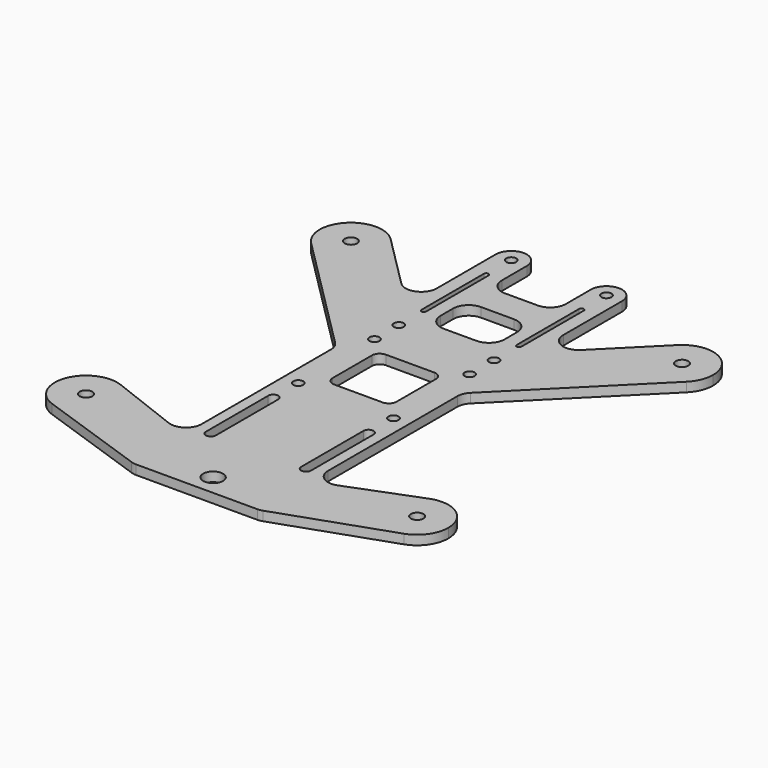
from build123d import *

# Parameters (mm, degrees)
F0_R      = 2
F0_R_2    = 1.6
F1_DEPTH  = 3
F3_R      = 1.6
F4_DEPTH  = 25
F6_DEPTH  = 25
F7_R      = 3.175
F8_DEPTH  = 25
F10_DEPTH = 25
F12_DEPTH = 25
F14_DEPTH = 3.001


# Not quite as in the source:
# - a pattern or mirror of a feature is missing from the dataset's text; its kind, count and spacing are read off the source's solid


with BuildPart() as f1:
    # F0 (on Top) → F1 (new body)
    with BuildSketch(Plane.XY):
        with BuildLine():
            ThreePointArc((60.1040764009, 45.9619407771), (62.2718039141, 49.2061742653), (63.033008589, 53.033008589))
            ThreePointArc((63.033008589, 53.033008589), (56.8598429126, 62.2718039141), (45.9619407771, 60.1040764009))
            ThreePointArc((45.9619407771, 60.1040764009), (45.9619407771, 45.9619407771), (60.1040764009, 45.9619407771))
        make_face()
        with Locations((53.033008589, 53.033008589)):
            Circle(F0_R, mode=Mode.SUBTRACT)
        with BuildLine():
            ThreePointArc((60.1040764009, 45.9619407771), (45.9619407771, 45.9619407771), (45.9619407771, 60.1040764009))
            Line((45.9619407771, 60.1040764009), (28.7855339059, 42.9276695297))
            ThreePointArc((28.7855339059, 42.9276695297), (23.3365828382, 41.843805773), (20.25, 46.4632034356))
            Line((20.25, 46.4632034356), (20.25, 70))
            ThreePointArc((20.25, 70), (18.7855339059, 73.5355339059), (15.25, 75))
            Line((15.25, 75), (0, 75))
            Line((0, 75), (0, 10.461255908))
            Line((0, 10.461255908), (7.75, 10.461255908))
            ThreePointArc((7.75, 10.461255908), (9.517766953, 9.729022861), (10.25, 7.961255908))
            Line((10.25, 7.961255908), (10.25, -7.75))
            ThreePointArc((10.25, -7.75), (9.517766953, -9.517766953), (7.75, -10.25))
            Line((7.75, -10.25), (0, -10.25))
            Line((0, -10.25), (0, -75))
            Line((0, -75), (19.4067466501, -75))
            ThreePointArc((19.4067466501, -75), (20.2382575597, -74.9303741853), (21.0466106195, -74.7234358429))
            Line((21.0466106195, -74.7234358429), (56.3127356997, -62.4798805623))
            ThreePointArc((56.3127356997, -62.4798805623), (43.6452735158, -56.4783576564), (49.4231031357, -43.7073138364))
            Line((49.4231031357, -43.7073138364), (27.0549527266, -52.3658545976))
            ThreePointArc((27.0549527266, -52.3658545976), (22.4237625395, -51.8276140894), (20.25, -47.7030072213))
            Line((20.25, -47.7030072213), (20.25, 4.0367965644))
            ThreePointArc((20.25, 4.0367965644), (20.6306023374, 5.9502137262), (21.7144660941, 7.5723304703))
            Line((21.7144660941, 7.5723304703), (60.1040764009, 45.9619407771))
        make_face()
        with Locations((15.25, -15.25)):
            Circle(F0_R_2, mode=Mode.SUBTRACT)
        with Locations((15.25, 15.25)):
            Circle(F0_R_2, mode=Mode.SUBTRACT)
        with BuildLine():
            ThreePointArc((63.033008589, -53.033008589), (58.6854835101, -44.7837948527), (49.4231031357, -43.7073138364))
            ThreePointArc((49.4231031357, -43.7073138364), (43.6452735158, -56.4783576564), (56.3127356997, -62.4798805623))
            ThreePointArc((56.3127356997, -62.4798805623), (61.181544381, -58.829676981), (63.033008589, -53.033008589))
        make_face()
        with Locations((53.033008589, -53.033008589)):
            Circle(F0_R, mode=Mode.SUBTRACT)
    extrude(amount=F1_DEPTH)

    # F2: F1 across plane


with BuildPart() as f1_1:
    add(f1.part)
    add(f1.part.mirror(Plane.YZ))

    # F3 (on face) → F4 (cut)
    with BuildSketch(Plane.XY.offset(3)):
        with Locations((15.25, 70)):
            Circle(F3_R)
        with Locations((15.25, 25)):
            Circle(F3_R)
    f4 = extrude(amount=-F4_DEPTH, mode=Mode.SUBTRACT)

    # F4_copies: F4 across plane
    add(f4.mirror(Plane(origin=(0, 0, 0), x_dir=(0, 0, -1), z_dir=(-1, 0, 0))), mode=Mode.SUBTRACT)

    # F5 (on face) → F6 (cut)
    with BuildSketch(Plane.XY.offset(3)):
        with BuildLine():
            Line((16.8499999975, -50.2499110026), (16.8486131231, -25.3166039246))
            ThreePointArc((16.8486131231, -25.3166039246), (15.2833091812, -23.6503467568), (13.65, -25.25))
            Line((13.65, -25.25), (13.65, -50.25))
            ThreePointArc((13.65, -50.25), (15.2500444987, -51.8499999994), (16.8499999975, -50.2499110026))
        make_face()
    f6 = extrude(amount=-F6_DEPTH, mode=Mode.SUBTRACT)

    # F6_copies: F6 across plane
    add(f6.mirror(Plane(origin=(0, 0, 0), x_dir=(0, 0, -1), z_dir=(-1, 0, 0))), mode=Mode.SUBTRACT)

    # F7 (on face) → F8 (cut)
    with BuildSketch(Plane.XY.offset(3)):
        with Locations((0, -68.425)):
            Circle(F7_R)
    extrude(amount=-F8_DEPTH, mode=Mode.SUBTRACT)

    # F9 (on face) → F10 (cut)
    with BuildSketch(Plane.XY.offset(3)):
        with BuildLine():
            ThreePointArc((-10.25, 60), (-8.7855339059, 56.4644660941), (-5.25, 55))
            Line((-5.25, 55), (5.25, 55))
            ThreePointArc((5.25, 55), (8.7855339059, 56.4644660941), (10.25, 60))
            Line((10.25, 60), (10.25, 70))
            ThreePointArc((10.25, 70), (11.7144660941, 73.5355339059), (15.25, 75))
            Line((15.25, 75), (15.25, 79.1207849979))
            Line((15.25, 79.1207849979), (-15.25, 79.1207849979))
            Line((-15.25, 79.1207849979), (-15.25, 75))
            ThreePointArc((-15.25, 75), (-11.7144660941, 73.5355339059), (-10.25, 70))
            Line((-10.25, 70), (-10.25, 60))
        make_face()
    extrude(amount=-F10_DEPTH, mode=Mode.SUBTRACT)

    # F11 (on face) → F12 (cut)
    with BuildSketch(Plane.XY.offset(3)):
        with BuildLine():
            ThreePointArc((10.25, 40.461255908), (8.7855339059, 43.9967898139), (5.25, 45.461255908))
            Line((5.25, 45.461255908), (-5.25, 45.461255908))
            ThreePointArc((-5.25, 45.461255908), (-8.7855339059, 43.9967898139), (-10.25, 40.461255908))
            Line((-10.25, 40.461255908), (-10.25, 35.461255908))
            ThreePointArc((-10.25, 35.461255908), (-8.7855339059, 31.9257220021), (-5.25, 30.461255908))
            Line((-5.25, 30.461255908), (5.25, 30.461255908))
            ThreePointArc((5.25, 30.461255908), (8.7855339059, 31.9257220021), (10.25, 35.461255908))
            Line((10.25, 35.461255908), (10.25, 40.461255908))
        make_face()
    extrude(amount=-F12_DEPTH, mode=Mode.SUBTRACT)

    # F13 (on face) → F14 (cut, through all)
    with BuildSketch(Plane.XY.offset(3)):
        with BuildLine():
            Line((-14.5, 35.0000002275), (-14.5, 60.0000002275))
            ThreePointArc((-14.5, 60.0000002275), (-15.222352045, 60.7494904479), (-15.9979615749, 60.0552585525))
            Line((-15.9979615749, 60.0552585525), (-15.9979615749, 59.9447419024))
            Line((-15.9979615749, 59.9447419024), (-15.9979615749, 35.0552585525))
            Line((-15.9979615749, 35.0552585525), (-15.9979615749, 34.9447419024))
            ThreePointArc((-15.9979615749, 34.9447419024), (-15.222352045, 34.250510007), (-14.5, 35.0000002275))
        make_face()
        with BuildLine():
            Line((-15.9979615749, 59.9447419024), (-15.9979615749, 60.0552585525))
            ThreePointArc((-15.9979615749, 60.0552585525), (-16, 60.0000002275), (-15.9979615749, 59.9447419024))
        make_face()
        with BuildLine():
            ThreePointArc((-15.9979615749, 35.0552585525), (-16, 35.0000002275), (-15.9979615749, 34.9447419024))
            Line((-15.9979615749, 34.9447419024), (-15.9979615749, 35.0552585525))
        make_face()
    f14 = extrude(amount=-F14_DEPTH, mode=Mode.SUBTRACT)

    # F14_copies: F14 across plane
    add(f14.mirror(Plane(origin=(0, 0, 0), x_dir=(0, 0, 1), z_dir=(1, 0, 0))), mode=Mode.SUBTRACT)


solid = f1_1.part
